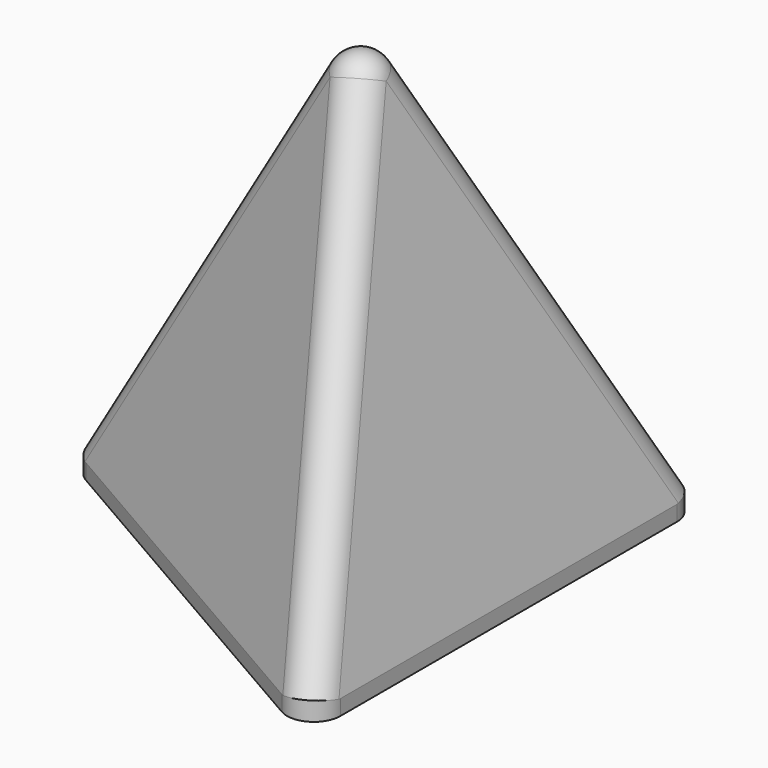
from build123d import *

# Parameters (mm, degrees)
F2_DEPTH     = 38.1
F4_T1_DEPTH  = 1620.39257698
F4_T3_DEPTH  = 3333.6434925305
F4_T5_DEPTH  = 3333.6434925305
F4_T7_DEPTH  = 3333.6434925305
F4_T12_DEPTH = 563.5574853852


# Not quite as in the source:
# - a fillet or chamfer that OpenCascade refuses, or shapes differently, is made with other operations: its cross-section is extruded or revolved along the edge and cut away or added


with BuildPart() as f2:
    # F0 (on Top) → F2 (new body, symmetric)
    with BuildSketch(Plane.XY):
        Polygon((733.2348418708, -1270), (733.2348418708, 1270), (-1466.4696837416, 0), align=None)
    extrude(amount=F2_DEPTH, both=True)

    # F2_face (on face) → F3 section 0
    with BuildSketch(Plane.XY.offset(38.1), mode=Mode.PRIVATE) as f3_s0:
        Polygon((-1466.4696837416, 0), (733.2348418708, -1270), (733.2348418708, 1270), align=None)
    loft([f3_s0.sketch, Vertex(0, 0, 2540)])

    # F4: fillet of radius 132.08 on 6 edges, made by hand

    # F4_s2 → F4_t1 (cut)
    with BuildSketch(Plane.XY.offset(-610.0231766592)):
        with BuildLine():
            ThreePointArc((535.1148418708, -1155.6153646682), (667.1948418708, -1155.6153646682), (733.2348418708, -1041.2307293363))
            Line((733.2348418708, -1041.2307293363), (733.2348418708, -1270))
            Line((733.2348418708, -1270), (535.1148418708, -1155.6153646682))
        make_face()
        with BuildLine():
            ThreePointArc((-1268.3496837416, -114.3846353318), (-1334.3896837416, 0), (-1268.3496837416, 114.3846353318))
            Line((-1268.3496837416, 114.3846353318), (-1466.4696837416, 0))
            Line((-1466.4696837416, 0), (-1268.3496837416, -114.3846353318))
        make_face()
        with BuildLine():
            ThreePointArc((733.2348418708, 1041.2307293363), (667.1948418708, 1155.6153646682), (535.1148418708, 1155.6153646682))
            Line((535.1148418708, 1155.6153646682), (733.2348418708, 1270))
            Line((733.2348418708, 1270), (733.2348418708, 1041.2307293363))
        make_face()
    extrude(amount=F4_T1_DEPTH, mode=Mode.SUBTRACT)

    # F4_s4 → F4_t3 (cut)
    with BuildSketch(Plane(origin=(391.2659726275, -677.6925438636, -1335.0543114113), x_dir=(-0.8660254038, -0.5, 0), z_dir=(-0.2528390453, 0.4379300726, 0.8627222431))):
        with BuildLine():
            ThreePointArc((109.7677163708, 1120.3987833195), (0, 1179.0201225453), (-109.7677163708, 1120.3987833195))
            Line((-109.7677163708, 1120.3987833195), (0, 1284.4223501838))
            Line((0, 1284.4223501838), (109.7677163708, 1120.3987833195))
        make_face()
    extrude(amount=F4_T3_DEPTH, mode=Mode.SUBTRACT)

    # F4_s6 → F4_t5 (cut)
    with BuildSketch(Plane(origin=(-782.5319452549, 0, -1335.0543114113), x_dir=(0, 1, 0), z_dir=(0.5056780906, 0, 0.8627222431))):
        with BuildLine():
            ThreePointArc((-109.7677163708, 1120.3987833195), (0, 1179.0201225453), (109.7677163708, 1120.3987833195))
            Line((109.7677163708, 1120.3987833195), (0, 1284.4223501838))
            Line((0, 1284.4223501838), (-109.7677163708, 1120.3987833195))
        make_face()
    extrude(amount=F4_T5_DEPTH, mode=Mode.SUBTRACT)

    # F4_s8 → F4_t7 (cut)
    with BuildSketch(Plane(origin=(391.2659726275, 677.6925438636, -1335.0543114113), x_dir=(0.8660254038, -0.5, 0), z_dir=(-0.2528390453, -0.4379300726, 0.8627222431))):
        with BuildLine():
            ThreePointArc((109.7677163708, 1120.3987833195), (0, 1179.0201225453), (-109.7677163708, 1120.3987833195))
            Line((-109.7677163708, 1120.3987833195), (0, 1284.4223501838))
            Line((0, 1284.4223501838), (109.7677163708, 1120.3987833195))
        make_face()
    extrude(amount=F4_T7_DEPTH, mode=Mode.SUBTRACT)


with BuildPart() as f4_tool10:
    # F4_s11 → F4_t12 (new body)
    with BuildSketch(Plane.XY.offset(2070.368762179)):
        Polygon((-769.8338415291, -206.2763561439), (206.2763561439, -769.8338415291), (769.8338415291, 206.2763561439), (-206.2763561439, 769.8338415291), align=None)
    extrude(amount=F4_T12_DEPTH)

    split(bisect_by=Plane(origin=(-451.6092654337, 782.2101929001, 1540.9540800131), x_dir=(-0.8660254038, -0.5, 0), z_dir=(-0.2528390453, 0.4379300726, 0.8627222431)), keep=Keep.TOP)

    split(bisect_by=Plane(origin=(-451.6092654337, -782.2101929001, 1540.9540800131), x_dir=(0.8660254038, -0.5, 0), z_dir=(-0.2528390453, -0.4379300726, 0.8627222431)), keep=Keep.TOP)

    split(bisect_by=Plane(origin=(903.2185308674, 0, 1540.9540800131), x_dir=(0, 1, 0), z_dir=(0.5056780906, 0, 0.8627222431)), keep=Keep.TOP)

    split(bisect_by=Plane(origin=(-342.7604796014, -593.6785654963, 200.9064519446), x_dir=(-0.8660254038, 0.5, 0), z_dir=(0.4798184479, 0.8310699301, -0.2812419391)), keep=Keep.TOP)

    split(bisect_by=Plane(origin=(685.5209592028, 0, 200.9064519446), x_dir=(0, 1, 0), z_dir=(-0.9596368957, 0, -0.2812419391)), keep=Keep.TOP)

    split(bisect_by=Plane(origin=(-342.7604796014, 593.6785654963, 200.9064519446), x_dir=(0.8660254038, 0.5, 0), z_dir=(0.4798184479, -0.8310699301, -0.2812419391)), keep=Keep.TOP)

    # F4_s19 → F4_t20 (revolve, cut)
    with BuildSketch(Plane(origin=(0, 0, 2070.368762179), x_dir=(0, 0, -1), z_dir=(-0.5, -0.8660254038, 0))):
        with BuildLine():
            ThreePointArc((0, -132.08), (132.08, 0), (0, 132.08))
            Line((0, 132.08), (0, -132.08))
        make_face()
    revolve(axis=Axis((0, 0, 2070.368762179), (0.8660254038, -0.5, 0)), mode=Mode.SUBTRACT)


with BuildPart() as f2_1:
    add(f2.part)

    # F4_t9: cut F4_tool10
    add(f4_tool10.part, mode=Mode.SUBTRACT)


solid = f2_1.part
